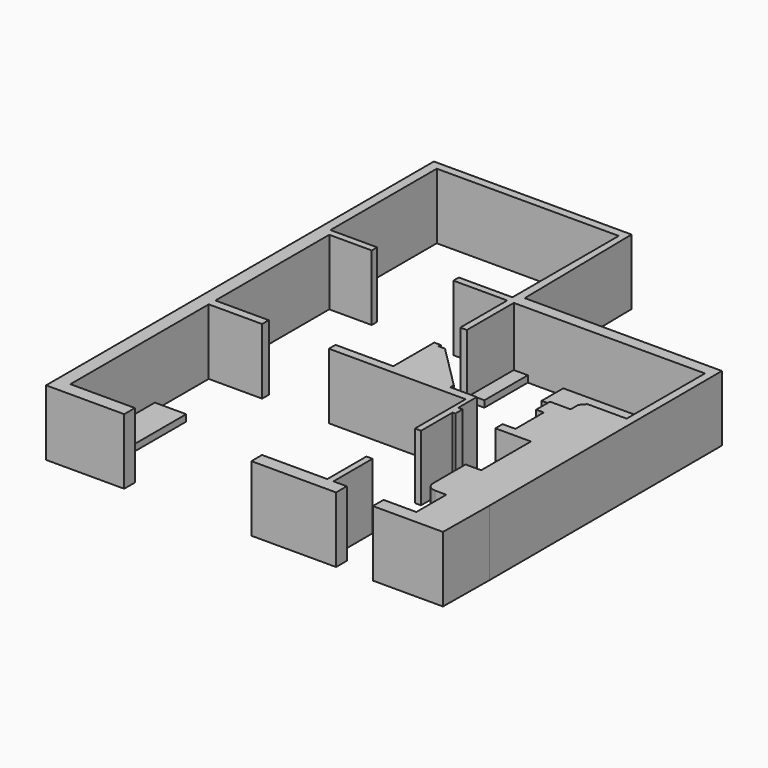
from build123d import *

# Parameters (mm, degrees)
F2_DEPTH = 254
F3_DEPTH = 25.4
F1_W     = 121.5051418
F1_H     = 291.3972582
F4_DEPTH = 25.4


# Not quite as in the source:
# - ends of sketch curves that miss each other by under 0.0002 mm in the source are joined


with BuildPart() as f2:
    # F1 (on face) → F2 (new body)
    with BuildSketch(Plane.XY):
        with BuildLine():
            Line((313.5800008442, -946.2826725998), (313.5800008442, -1103.1705731998))
            ThreePointArc((313.5800008442, -1103.1705731998), (323.4993407748, -1127.1179168691), (347.4466844442, -1137.0372313998))
            Line((347.4466844442, -1137.0372313998), (391.6476882442, -1137.0372567998))
            Line((391.6476882442, -1137.0372567998), (391.6476882442, -1281.7658725998))
            Line((391.6476882442, -1281.7658725998), (264.6476882442, -1281.7658725998))
            Line((264.6476882442, -1281.7658725998), (264.6476882442, -1333.3786725998))
            Line((264.6476882442, -1333.3786725998), (535.6998512442, -1333.3786725998))
            Line((535.6998512442, -1333.3786725998), (538.0177605074, -1111.6484430823))
            Line((538.0177605074, -1111.6484430823), (535.9808760803, 14.9786700639))
            Line((535.9808760803, 14.9786700639), (-226.6753639778, 14.9786700639))
            Line((-226.6753639778, 14.9786700639), (-234.6419504656, 541.2551566362))
            Line((-234.6419504656, 541.2551566362), (-999.1706609726, 541.2551566362))
            Line((-999.1706609726, 541.2551566362), (-999.1706609726, -1333.3786725998))
            Line((-999.1706609726, -1333.3786725998), (-697.0301953558, -1333.3786725998))
            Line((-697.0301953558, -1333.3786725998), (-697.0301953558, -1281.7658725998))
            Line((-697.0301953558, -1281.7658725998), (-946.4920535558, -1281.7658725998))
            Line((-946.4920535558, -1281.7658725998), (-946.4920535558, -1164.9343561998))
            Line((-946.4920535558, -1164.9343561998), (-946.4920535558, -873.5370979998))
            Line((-946.4920535558, -873.5370979998), (-946.4920535558, -612.9500143998))
            Line((-946.4920535558, -612.9500143998), (-740.0408535558, -612.9500143998))
            Line((-740.0408535558, -612.9500143998), (-740.0408535558, -587.1436143998))
            Line((-740.0408535558, -587.1436143998), (-740.0408535558, -580.7766725998))
            Line((-740.0408535558, -580.7766725998), (-946.4920535558, -580.7766725998))
            Line((-946.4920535558, -580.7766725998), (-946.4920535558, -30.2401307998))
            Line((-946.4920535558, -30.2401307998), (-782.2387117558, -30.2401307998))
            Line((-782.2387117558, -30.2401307998), (-782.2387117558, -3.9934725998))
            Line((-782.2387117558, -3.9934725998), (-962.8835117558, -3.9934725998))
            Line((-962.8835117558, -3.9934725998), (-962.8835117558, 510.0225682002))
            Line((-962.8835117558, 510.0225682002), (-259.0749117558, 510.0225682002))
            Line((-259.0749117558, 510.0225682002), (-259.0749117558, -3.9934725998))
            Line((-259.0749117558, -3.9934725998), (-466.6013953558, -3.9934725998))
            Line((-466.6013953558, -3.9934725998), (-466.6013953558, -30.2401307998))
            Line((-466.6013953558, -30.2401307998), (-258.3213953558, -30.2401307998))
            Line((-258.3213953558, -30.2401307998), (-258.3213953558, -257.1468143998))
            Line((-258.3213953558, -257.1468143998), (-232.9213953558, -257.1468143998))
            Line((-232.9213953558, -257.1468143998), (-232.9213953558, -240.0117203998))
            Line((-232.9213953558, -240.0117203998), (-232.9213953558, -30.0735575998))
            Line((-232.9213953558, -30.0735575998), (-178.7347117587, -30.0383741748))
            Line((-178.7347117587, -30.0383741748), (-41.5747117624, -29.9493161581))
            Line((-41.5747117624, -29.9493161581), (506.0763646442, -29.5937261998))
            Line((506.0763646442, -29.5937261998), (506.0763646442, -408.2670861998))
            Line((506.0763646442, -408.2670861998), (380.8600796442, -408.2670861998))
            Line((380.8600796442, -408.2670861998), (354.5230482442, -408.2670861998))
            Line((354.5230482442, -408.2670861998), (335.9305276442, -429.1228229998))
            Line((335.9305276442, -429.1228229998), (335.9305276442, -466.3761647998))
            Line((335.9305276442, -466.3761647998), (256.0446066442, -466.3761647998))
            Line((256.0446066442, -466.3761647998), (256.0446066442, -533.2095337998))
            Line((256.0446066442, -533.2095337998), (285.5676616442, -533.2095337998))
            Line((285.5676616442, -533.2095337998), (285.5676616442, -670.3695337998))
            Line((285.5676616442, -670.3695337998), (236.1608008442, -670.3695337998))
            Line((236.1608008442, -670.3695337998), (236.1608008442, -705.4229307998))
            Line((236.1608008442, -705.4229307998), (373.7949426442, -705.4229307998))
            Line((373.7949426442, -705.4229307998), (373.7949426442, -946.2826725998))
            Line((373.7949426442, -946.2826725998), (313.5800008442, -946.2826725998))
        make_face()
    extrude(amount=F2_DEPTH)


with BuildPart() as f2b:
    # F1 (on face) → F2, piece 2 (new body)
    with BuildSketch(Plane.XY):
        Polygon((-258.3213953558, -382.6566725998), (-258.3213953558, -580.7766725998), (-481.9768535558, -580.7766725998), (-481.9768535558, -612.9500143998), (47.0543464442, -612.9500143998), (47.0543464442, -858.1108143998), (70.7610046442, -858.1108143998), (70.7610046442, -705.4229307998), (81.3224008442, -705.4229307998), (81.3224008442, -670.3695337998), (64.3890844442, -670.3695337998), (64.3890844442, -580.6228501998), (-38.0575991558, -580.6228501998), (-38.0575991558, -563.6895337998), (-208.0837767558, -393.6633307998), (-232.9213953558, -393.6633307998), (-232.9213953558, -382.6566725998), align=None)
    extrude(amount=F2_DEPTH)


with BuildPart() as f2c:
    # F1 (on face) → F2, piece 3 (new body)
    with BuildSketch(Plane.XY):
        Polygon((-205.2032135558, -1333.3786725998), (122.4076882442, -1333.3786725998), (122.4076882442, -1281.7658725998), (70.7610046442, -1281.7658725998), (70.7610046442, -1092.5189307998), (47.0543464442, -1092.5189307998), (47.0543464442, -1281.7658725998), (-205.2032135558, -1281.7658725998), align=None)
    extrude(amount=F2_DEPTH)


with BuildPart() as f3:
    # F1 (on face) → F3 (new body)
    with BuildSketch(Plane.XY):
        Polygon((380.8600796442, -274.4937443998), (380.8600796442, -408.2670861998), (506.0763646442, -408.2670861998), (506.0763646442, -29.5937261998), (-41.5747117624, -29.9493161581), (-41.5747117558, -134.9359843998), (339.4252882442, -134.9359843998), (401.0897064442, -196.6004025998), (401.0897064442, -274.4937443998), align=None)
    extrude(amount=F3_DEPTH)


with BuildPart() as f3b:
    # F1 (on face) → F3, piece 2 (new body)
    with BuildSketch(Plane.XY):
        Polygon((-178.7347117558, -240.0117203998), (-178.7347117558, -30.0383785998), (-232.9213953558, -30.0735575998), (-232.9213953558, -240.0117203998), align=None)
    extrude(amount=F3_DEPTH)


with BuildPart() as f4:
    # F1 (on face) → F4 (new body)
    with BuildSketch(Plane.XY):
        with Locations((-885.7394826558, -1019.2357270998)):
            Rectangle(F1_W, F1_H)
    extrude(amount=F4_DEPTH)


solid = Compound([f2.part, f2b.part, f2c.part, f3.part, f3b.part, f4.part])
